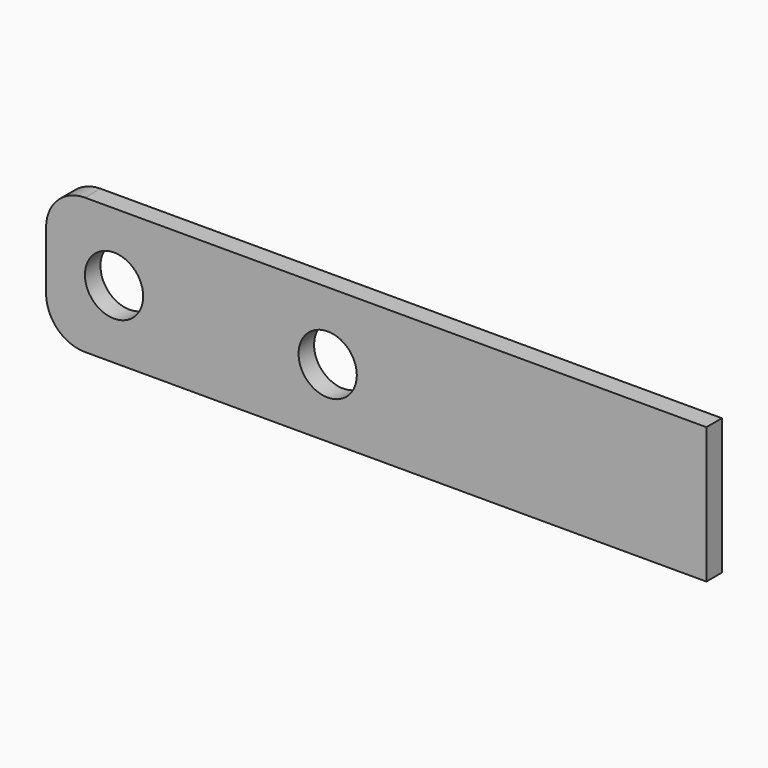
from build123d import *

# Parameters (mm, degrees)
F0_W          = 340
F0_H          = 70
F1_DEPTH      = 10
F2_R          = 20
F3_R          = 15
F4_DEPTH      = 353
F4_DEPTH_BACK = 25


# Not quite as in the source:
# - an extrude ends at something that could not be found from the text; its depth is read off the source's solid


with BuildPart() as f1:
    # F0 (on Front) → F1 (new body)
    with BuildSketch(Plane.XZ):
        Rectangle(F0_W, F0_H)
    extrude(amount=F1_DEPTH)

    # F2
    f2_edges = [f1.edges().sort_by_distance(p)[0] for p in [
        (-170, -5, 35),
        (-170, -5, -35),
    ]]
    fillet(f2_edges, radius=F2_R)

    # F3 (on Front) → F4 (cut, two sides)
    with BuildSketch(Plane.XZ) as f4_sk:
        with Locations((-135, 0)):
            Circle(F3_R)
        with Locations((-25, 0)):
            Circle(F3_R)
    extrude(amount=-F4_DEPTH, mode=Mode.SUBTRACT)
    extrude(f4_sk.sketch, amount=F4_DEPTH_BACK, mode=Mode.SUBTRACT)


solid = f1.part
